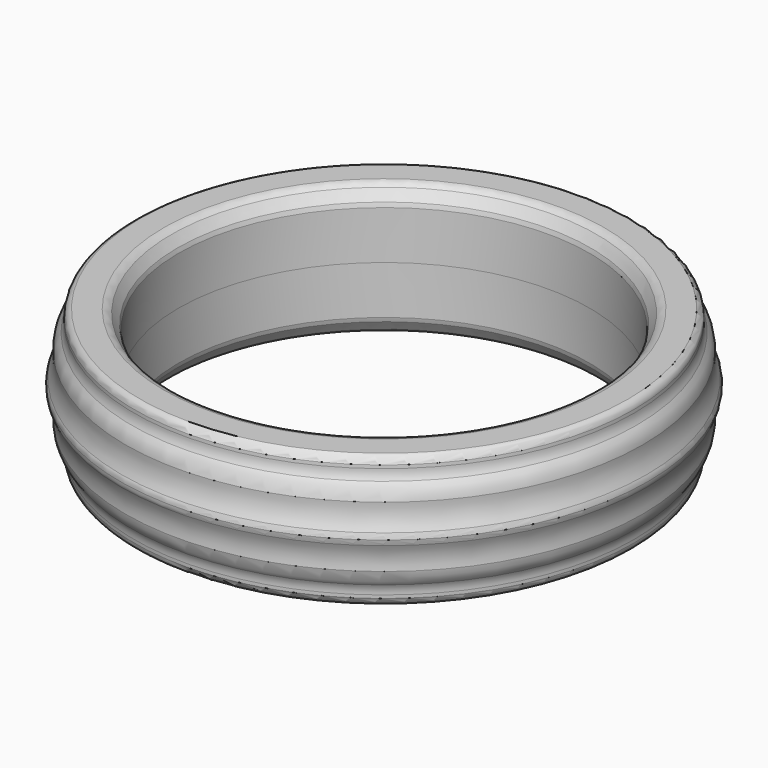
from build123d import *

# Parameters (mm, degrees)
F2_R = 0.4


# Not quite as in the source:
# - a feature names something its author has since deleted; it is built from what else it names


with BuildPart() as f1:
    # F0 (on Front) → F1 (revolve)
    with BuildSketch(Plane.XZ):
        with BuildLine():
            Line((9, 2.2145714873), (9, 0))
            Line((9, 0), (11.007581126, 1e-10))
            Line((11.007581126, 1e-10), (11.557581126, 1e-10))
            ThreePointArc((11.557581126, 1e-10), (11.5428486774, 0.1264462272), (11.4994405865, 0.2461184088))
            ThreePointArc((11.4994405865, 0.2461184088), (11.3275404558, 0.776753068), (11.320879477, 1.3344971203))
            ThreePointArc((11.320879477, 1.3344971203), (11.2446825964, 1.6904409043), (11.0480292202, 1.9967567406))
            ThreePointArc((11.0480292202, 1.9967567406), (10.9658405694, 2.2081954603), (10.9457389311, 2.4341539314))
            Line((10.9457389311, 2.4341539314), (10.9411267847, 2.5725573716))
            ThreePointArc((10.9411267847, 2.5725573716), (10.8685098139, 2.774597304), (10.6915943502, 2.8962290327))
            Line((10.6915943502, 2.8962290327), (9.4479103732, 2.8962290327))
            add(Edge.make_bspline(
                [(9.4479103732, 2.8962290327), (9.1998794596, 2.6115665992), (9, 2.2145714873)],
                knots=[4.1109906217, 4.1109906217, 4.1109906217, 4.7361224927, 4.7361224927, 4.7361224927], degree=2, weights=[1, 0.9515476749, 1]))
        make_face()
    revolve(axis=Axis((0, 0, 0.9835734963), (0, 0, 1)))

    # F2
    f2_edges = [f1.edges().sort_by_distance(p)[0] for p in [
        (-9, 0, 2.214571),
        (-9.44791, 0, 2.896229),
    ]]
    fillet(f2_edges, radius=F2_R)

    # F3: F1 across plane


with BuildPart() as f1_1:
    add(f1.part)
    add(f1.part.mirror(Plane.XY))


solid = f1_1.part
